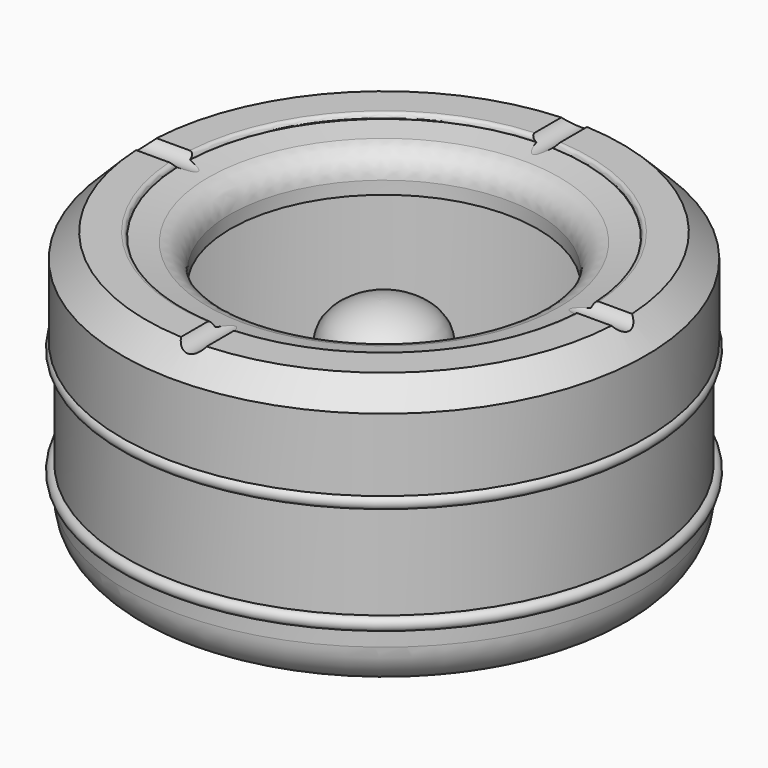
from build123d import *

# Parameters (mm, degrees)
F5_R          = 6
F6_R          = 1
F7_DEPTH      = 61.5010001
F7_DEPTH_BACK = 61.5010001
F9_DEPTH      = 61.5010001
F9_DEPTH_BACK = 61.5010001


# Not quite as in the source:
# - a feature names something its author has since deleted; it is built from what else it names


with BuildPart() as f1:
    # F0 (on Front) → F1 (revolve)
    with BuildSketch(Plane.XZ):
        with BuildLine():
            add(Edge.make_bspline(
                [(-12.6650770704, 42.5924675862), (-11.9824642458, 46.4632037959), (-6.2790805461, 50), (0, 50)],
                knots=[0, 0, 0, 0, 14.6722770441, 14.6722770441, 14.6722770441, 14.6722770441], degree=3))
            Line((-12.6650770704, 42.5924675862), (-20, 1))
            Line((-20, 1), (-50, 1))
            ThreePointArc((-50, 1), (-56.3639610307, 3.6360389693), (-59, 10))
            Line((-59, 10), (-59, 50))
            Line((-59, 50), (-60, 50))
            Line((-60, 50), (-60, 41.5))
            ThreePointArc((-60, 41.5), (-61.5, 40), (-60, 38.5))
            Line((-60, 38.5), (-60, 16.5))
            ThreePointArc((-60, 16.5), (-61.5, 15), (-60, 13.5))
            Line((-60, 13.5), (-60, 10))
            ThreePointArc((-60, 10), (-57.0710678119, 2.9289321881), (-50, 0))
            Line((-50, 0), (0, 0))
            Line((0, 0), (0, 50))
        make_face()
    revolve(axis=Axis((0, 0, 3.8219820102), (0, 0, -1)))


with BuildPart() as f3:
    # F2 (on Front) → F3 (revolve)
    with BuildSketch(Plane.XZ):
        Polygon((-61, 41.5), (-60, 41.5), (-60, 57.6322230848), (-36.8035080135, 57.6322230848), (-36.8035080135, 52.9242841807), (-35.8035080135, 52.9242841807), (-35.8035080135, 61.0642433167), (-46.7573593129, 62.7709701657), (-46.7573593129, 63.9313480565), (-55.4644660941, 63.9313480565), (-61, 58.3958141506), align=None)
    revolve(axis=Axis((0, 0, 92.2469310462), (0, 0, -1)))

    # F5
    f5_edges = [f3.edges().sort_by_distance(p)[0] for p in [
        (35.803508, 0, 61.064243),
    ]]
    fillet(f5_edges, radius=F5_R)

    # F6
    f6_edges = [f3.edges().sort_by_distance(p)[0] for p in [
        (46.757359, 0, 63.931348),
    ]]
    fillet(f6_edges, radius=F6_R)

    # F4 (on Front) → F7 (cut, two sides)
    with BuildSketch(Plane.XZ) as f7_sk:
        with BuildLine():
            Line((3, 63.9313480565), (-3, 63.9313480565))
            ThreePointArc((-3, 63.9313480565), (0, 62.2341236942), (3, 63.9313480565))
        make_face()
    extrude(amount=-F7_DEPTH, mode=Mode.SUBTRACT)
    extrude(f7_sk.sketch, amount=F7_DEPTH_BACK, mode=Mode.SUBTRACT)

    # F8 (on Right) → F9 (cut, two sides)
    with BuildSketch(Plane.YZ) as f9_sk:
        with BuildLine():
            ThreePointArc((-3, 63.9313480565), (0, 62.2341236942), (3, 63.9313480565))
            Line((3, 63.9313480565), (-3, 63.9313480565))
        make_face()
    extrude(amount=F9_DEPTH, mode=Mode.SUBTRACT)
    extrude(f9_sk.sketch, amount=-F9_DEPTH_BACK, mode=Mode.SUBTRACT)


solid = Compound([f1.part, f3.part])
